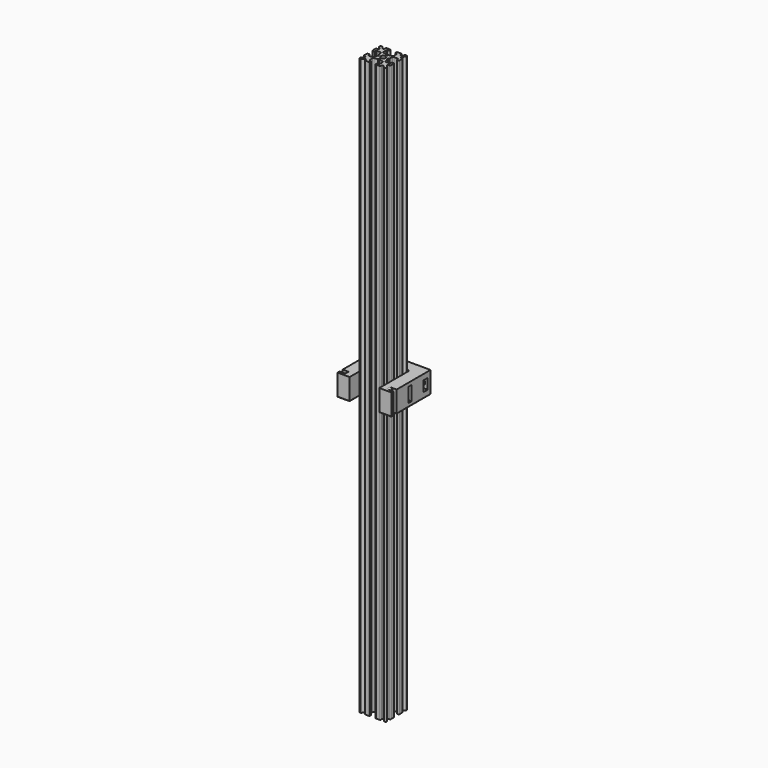
from build123d import *

# Parameters (mm, degrees)
F6_DEPTH  = 6
F7_DEPTH  = 160
F4_W      = 6
F4_H      = 2.8
F8_DEPTH  = 2.9
F11_DEPTH = 4
F12_R     = 1
F16_R     = 1.5
F13_SIZE  = 0.25


# Not quite as in the source:
# - a feature of the source that left no trace in its solid (it failed there, or was rolled back) is left out


with BuildPart() as f6:
    # F2 (on Top) → F6 (new body, symmetric)
    with BuildSketch(Plane.XY):
        Polygon((0, 14.1908953894), (-15, 14.1908953894), (-15, -9.4), (-12.8, -9.4), (-12.8, -11.6), (-15, -11.6), (-15, -13), (-8.25, -13), (-8.25, -8), (-8.25, 8), (8.25, 8), (8.25, -8), (8.25, -13), (15, -13), (15, -11.6), (12.8, -11.6), (12.8, -9.4), (15, -9.4), (15, 14.1908953894), align=None)
    extrude(amount=F6_DEPTH, both=True)

    # F4 (on Top) → F8 (cut, symmetric)
    with BuildSketch(Plane.XY):
        with Locations((-12, 10.7908953894)):
            Rectangle(F4_W, F4_H)
        with Locations((12, 10.7908953894)):
            Rectangle(F4_W, F4_H)
    extrude(amount=F8_DEPTH, both=True, mode=Mode.SUBTRACT)

    # F5 (on Top) → F9 (revolve, cut)
    with BuildSketch(Plane.XY):
        Polygon((-12, 7.8908953894), (-12, 12.1908953894), (-12, 14.1908953894), (-13.6, 14.1908953894), (-13.6, 12.1908953894), (-13.6, 7.8908953894), align=None)
    revolve(axis=Axis((-12, 13.1908953894, 0), (0, 1, 0)), mode=Mode.SUBTRACT)

    # F5 (on Top) → F10 (revolve, cut)
    with BuildSketch(Plane.XY):
        Polygon((12, 14.1908953894), (12, 12.1908953894), (12, 7.8908953894), (13.6, 7.8908953894), (13.6, 12.1908953894), (13.6, 14.1908953894), align=None)
    revolve(axis=Axis((12, 13.1908953894, 0), (0, 1, 0)), mode=Mode.SUBTRACT)

    # F3 (on Top) → F11 (cut, symmetric)
    with BuildSketch(Plane.XY):
        with BuildLine():
            ThreePointArc((-10.0158953894, 3.275), (-11.9460022518, 2.6458103674), (-13.1344888224, 1))
            Line((-13.1344888224, 1), (-21.4828029275, 1))
            Line((-21.4828029275, 1), (-21.4828029275, -1))
            Line((-21.4828029275, -1), (-13.1344888224, -1))
            ThreePointArc((-13.1344888224, -1), (-11.9460022518, -2.6458103674), (-10.0158953894, -3.275))
            Line((-10.0158953894, -3.275), (-8.25, -3.275))
            Line((-8.25, -3.275), (-8.25, 0))
            Line((-8.25, 0), (-8.25, 3.275))
            Line((-8.25, 3.275), (-10.0158953894, 3.275))
        make_face()
        with BuildLine():
            ThreePointArc((-1, 13.1344888224), (-2.6458103674, 11.9460022518), (-3.275, 10.0158953894))
            Line((-3.275, 10.0158953894), (-3.275, 8.25))
            Line((-3.275, 8.25), (0, 8.25))
            Line((0, 8.25), (3.275, 8.25))
            Line((3.275, 8.25), (3.275, 10.0158953894))
            ThreePointArc((3.275, 10.0158953894), (2.6458103674, 11.9460022518), (1, 13.1344888224))
            Line((1, 13.1344888224), (1, 21.4828029275))
            Line((1, 21.4828029275), (-1, 21.4828029275))
            Line((-1, 21.4828029275), (-1, 13.1344888224))
        make_face()
        Polygon((0, 8.25), (-3.275, 8.25), (-3.275, 2.3650461808), (3.275, 2.3650461808), (3.275, 8.25), align=None)
        with BuildLine():
            ThreePointArc((13.1344888224, 1), (11.9460022518, 2.6458103674), (10.0158953894, 3.275))
            Line((10.0158953894, 3.275), (8.25, 3.275))
            Line((8.25, 3.275), (8.25, 0))
            Line((8.25, 0), (8.25, -3.275))
            Line((8.25, -3.275), (10.0158953894, -3.275))
            ThreePointArc((10.0158953894, -3.275), (11.9460022518, -2.6458103674), (13.1344888224, -1))
            Line((13.1344888224, -1), (21.4828029275, -1))
            Line((21.4828029275, -1), (21.4828029275, 1))
            Line((21.4828029275, 1), (13.1344888224, 1))
        make_face()
    extrude(amount=F11_DEPTH, both=True, mode=Mode.SUBTRACT)

    # F12
    f12_edges = [f6.edges().sort_by_distance(p)[0] for p in [
        (-8.25, 8, 0),
        (8.25, 8, 0),
    ]]
    fillet(f12_edges, radius=F12_R)

    # F16
    f16_edges = [f6.edges().sort_by_distance(p)[0] for p in [
        (12.8, -10.5, -6),
        (-12.8, -10.5, -6),
        (12.8, -10.5, 6),
        (-12.8, -10.5, 6),
    ]]
    fillet(f16_edges, radius=F16_R)

    # F13
    f13_edges = [f6.edges().sort_by_distance(p)[0] for p in [
        (12.05, -11.6, -6),
        (13.9, -11.6, -6),
        (11.3, -10.5, -6),
        (15, -12.3, -6),
        (12.05, -9.4, -6),
        (11.625, -13, -6),
        (13.9, -9.4, -6),
        (8.25, -3, -6),
        (15, 2.395448, -6),
        (7.957107, 7.707107, -6),
        (0, 14.190895, -6),
        (0, 8, -6),
        (-15, 2.395448, -6),
        (-7.957107, 7.707107, -6),
        (-13.9, -9.4, -6),
        (-8.25, -3, -6),
        (-12.05, -9.4, -6),
        (-11.625, -13, -6),
        (-11.3, -10.5, -6),
        (-15, -12.3, -6),
        (-12.05, -11.6, -6),
        (-13.9, -11.6, -6),
    ]]
    chamfer(f13_edges, length=F13_SIZE)


with BuildPart() as f7:
    # F0 (on Top) → F7 (new body, symmetric)
    with BuildSketch(Plane.XY):
        with BuildLine():
            Line((-7.5, -6.7171572875), (-7.5, -7))
            ThreePointArc((-7.5, -7), (-7.3535533906, -7.3535533906), (-7, -7.5))
            Line((-7, -7.5), (-6.7171572875, -7.5))
            ThreePointArc((-6.7171572875, -7.5), (-6.5258155713, -7.4619397663), (-6.3636038969, -7.3535533906))
            Line((-6.3636038969, -7.3535533906), (-5.2564971157, -6.2464466094))
            ThreePointArc((-5.2564971157, -6.2464466094), (-4.711602009, -6.1380602337), (-4.4029437252, -6.6))
            Line((-4.4029437252, -6.6), (-4.4029437252, -7))
            ThreePointArc((-4.4029437252, -7), (-4.2564971157, -7.3535533906), (-3.9029437252, -7.5))
            Line((-3.9029437252, -7.5), (-2.1, -7.5))
            ThreePointArc((-2.1, -7.5), (-1.7464466094, -7.3535533906), (-1.6, -7))
            Line((-1.6, -7), (-1.6, -6.6))
            ThreePointArc((-1.6, -6.6), (-1.7464466094, -6.2464466094), (-2.1, -6.1))
            Line((-2.1, -6.1), (-2.7, -6.1))
            ThreePointArc((-2.7, -6.1), (-2.8414213562, -6.0414213562), (-2.9, -5.9))
            Line((-2.9, -5.9), (-2.9, -3.7379295017))
            ThreePointArc((-2.9, -3.7379295017), (-2.7836336902, -3.4172658278), (-2.4886992329, -3.2458599476))
            Line((-2.4886992329, -3.2458599476), (-0.7345203068, -2.929656021))
            ThreePointArc((-0.7345203068, -2.929656021), (-0.6165465239, -2.8610936689), (-0.57, -2.7328281993))
            Line((-0.57, -2.7328281993), (-0.57, -2.6))
            ThreePointArc((-0.57, -2.6), (-0.5114213562, -2.4585786438), (-0.37, -2.4))
            Line((-0.37, -2.4), (0, -2.4))
            Line((0, -2.4), (0.37, -2.4))
            ThreePointArc((0.37, -2.4), (0.5114213562, -2.4585786438), (0.57, -2.6))
            Line((0.57, -2.6), (0.57, -2.7328281993))
            ThreePointArc((0.57, -2.7328281993), (0.6165465239, -2.8610936689), (0.7345203068, -2.929656021))
            Line((0.7345203068, -2.929656021), (2.4886992329, -3.2458599476))
            ThreePointArc((2.4886992329, -3.2458599476), (2.7836336902, -3.4172658278), (2.9, -3.7379295017))
            Line((2.9, -3.7379295017), (2.9, -5.9))
            ThreePointArc((2.9, -5.9), (2.8414213562, -6.0414213562), (2.7, -6.1))
            Line((2.7, -6.1), (2.1, -6.1))
            ThreePointArc((2.1, -6.1), (1.7464466094, -6.2464466094), (1.6, -6.6))
            Line((1.6, -6.6), (1.6, -7))
            ThreePointArc((1.6, -7), (1.7464466094, -7.3535533906), (2.1, -7.5))
            Line((2.1, -7.5), (3.9029437252, -7.5))
            ThreePointArc((3.9029437252, -7.5), (4.2564971157, -7.3535533906), (4.4029437252, -7))
            Line((4.4029437252, -7), (4.4029437252, -6.6))
            ThreePointArc((4.4029437252, -6.6), (4.711602009, -6.1380602337), (5.2564971157, -6.2464466094))
            Line((5.2564971157, -6.2464466094), (6.3636038969, -7.3535533906))
            ThreePointArc((6.3636038969, -7.3535533906), (6.5258155713, -7.4619397663), (6.7171572875, -7.5))
            Line((6.7171572875, -7.5), (7, -7.5))
            ThreePointArc((7, -7.5), (7.3535533906, -7.3535533906), (7.5, -7))
            Line((7.5, -7), (7.5, -6.7171572875))
            ThreePointArc((7.5, -6.7171572875), (7.4619397663, -6.5258155713), (7.3535533906, -6.3636038969))
            Line((7.3535533906, -6.3636038969), (6.2464466094, -5.2564971157))
            ThreePointArc((6.2464466094, -5.2564971157), (6.1380602337, -4.711602009), (6.6, -4.4029437252))
            Line((6.6, -4.4029437252), (7, -4.4029437252))
            ThreePointArc((7, -4.4029437252), (7.3535533906, -4.2564971157), (7.5, -3.9029437252))
            Line((7.5, -3.9029437252), (7.5, -2.1))
            ThreePointArc((7.5, -2.1), (7.3535533906, -1.7464466094), (7, -1.6))
            Line((7, -1.6), (6.6, -1.6))
            ThreePointArc((6.6, -1.6), (6.2464466094, -1.7464466094), (6.1, -2.1))
            Line((6.1, -2.1), (6.1, -2.7))
            ThreePointArc((6.1, -2.7), (6.0414213562, -2.8414213562), (5.9, -2.9))
            Line((5.9, -2.9), (3.7379295017, -2.9))
            ThreePointArc((3.7379295017, -2.9), (3.4172658278, -2.7836336902), (3.2458599476, -2.4886992329))
            Line((3.2458599476, -2.4886992329), (2.929656021, -0.7345203068))
            ThreePointArc((2.929656021, -0.7345203068), (2.8610936689, -0.6165465239), (2.7328281993, -0.57))
            Line((2.7328281993, -0.57), (2.6, -0.57))
            ThreePointArc((2.6, -0.57), (2.4585786438, -0.5114213562), (2.4, -0.37))
            Line((2.4, -0.37), (2.4, 0))
            Line((2.4, 0), (2.4, 0.37))
            ThreePointArc((2.4, 0.37), (2.4585786438, 0.5114213562), (2.6, 0.57))
            Line((2.6, 0.57), (2.7328281993, 0.57))
            ThreePointArc((2.7328281993, 0.57), (2.8610936689, 0.6165465239), (2.929656021, 0.7345203068))
            Line((2.929656021, 0.7345203068), (3.2458599476, 2.4886992329))
            ThreePointArc((3.2458599476, 2.4886992329), (3.4172658278, 2.7836336902), (3.7379295017, 2.9))
            Line((3.7379295017, 2.9), (5.9, 2.9))
            ThreePointArc((5.9, 2.9), (6.0414213562, 2.8414213562), (6.1, 2.7))
            Line((6.1, 2.7), (6.1, 2.1))
            ThreePointArc((6.1, 2.1), (6.2464466094, 1.7464466094), (6.6, 1.6))
            Line((6.6, 1.6), (7, 1.6))
            ThreePointArc((7, 1.6), (7.3535533906, 1.7464466094), (7.5, 2.1))
            Line((7.5, 2.1), (7.5, 3.9029437252))
            ThreePointArc((7.5, 3.9029437252), (7.3535533906, 4.2564971157), (7, 4.4029437252))
            Line((7, 4.4029437252), (6.6, 4.4029437252))
            ThreePointArc((6.6, 4.4029437252), (6.1380602337, 4.711602009), (6.2464466094, 5.2564971157))
            Line((6.2464466094, 5.2564971157), (7.3535533906, 6.3636038969))
            ThreePointArc((7.3535533906, 6.3636038969), (7.4619397663, 6.5258155713), (7.5, 6.7171572875))
            Line((7.5, 6.7171572875), (7.5, 7))
            ThreePointArc((7.5, 7), (7.3535533906, 7.3535533906), (7, 7.5))
            Line((7, 7.5), (6.7171572875, 7.5))
            ThreePointArc((6.7171572875, 7.5), (6.5258155713, 7.4619397663), (6.3636038969, 7.3535533906))
            Line((6.3636038969, 7.3535533906), (5.2564971157, 6.2464466094))
            ThreePointArc((5.2564971157, 6.2464466094), (4.711602009, 6.1380602337), (4.4029437252, 6.6))
            Line((4.4029437252, 6.6), (4.4029437252, 7))
            ThreePointArc((4.4029437252, 7), (4.2564971157, 7.3535533906), (3.9029437252, 7.5))
            Line((3.9029437252, 7.5), (2.1, 7.5))
            ThreePointArc((2.1, 7.5), (1.7464466094, 7.3535533906), (1.6, 7))
            Line((1.6, 7), (1.6, 6.6))
            ThreePointArc((1.6, 6.6), (1.7464466094, 6.2464466094), (2.1, 6.1))
            Line((2.1, 6.1), (2.7, 6.1))
            ThreePointArc((2.7, 6.1), (2.8414213562, 6.0414213562), (2.9, 5.9))
            Line((2.9, 5.9), (2.9, 3.7379295017))
            ThreePointArc((2.9, 3.7379295017), (2.7836336902, 3.4172658278), (2.4886992329, 3.2458599476))
            Line((2.4886992329, 3.2458599476), (0.7345203068, 2.929656021))
            ThreePointArc((0.7345203068, 2.929656021), (0.6165465239, 2.8610936689), (0.57, 2.7328281993))
            Line((0.57, 2.7328281993), (0.57, 2.6))
            ThreePointArc((0.57, 2.6), (0.5114213562, 2.4585786438), (0.37, 2.4))
            Line((0.37, 2.4), (0, 2.4))
            Line((0, 2.4), (-0.37, 2.4))
            ThreePointArc((-0.37, 2.4), (-0.5114213562, 2.4585786438), (-0.57, 2.6))
            Line((-0.57, 2.6), (-0.57, 2.7328281993))
            ThreePointArc((-0.57, 2.7328281993), (-0.6165465239, 2.8610936689), (-0.7345203068, 2.929656021))
            Line((-0.7345203068, 2.929656021), (-2.4886992329, 3.2458599476))
            ThreePointArc((-2.4886992329, 3.2458599476), (-2.7836336902, 3.4172658278), (-2.9, 3.7379295017))
            Line((-2.9, 3.7379295017), (-2.9, 5.9))
            ThreePointArc((-2.9, 5.9), (-2.8414213562, 6.0414213562), (-2.7, 6.1))
            Line((-2.7, 6.1), (-2.1, 6.1))
            ThreePointArc((-2.1, 6.1), (-1.7464466094, 6.2464466094), (-1.6, 6.6))
            Line((-1.6, 6.6), (-1.6, 7))
            ThreePointArc((-1.6, 7), (-1.7464466094, 7.3535533906), (-2.1, 7.5))
            Line((-2.1, 7.5), (-3.9029437252, 7.5))
            ThreePointArc((-3.9029437252, 7.5), (-4.2564971157, 7.3535533906), (-4.4029437252, 7))
            Line((-4.4029437252, 7), (-4.4029437252, 6.6))
            ThreePointArc((-4.4029437252, 6.6), (-4.711602009, 6.1380602337), (-5.2564971157, 6.2464466094))
            Line((-5.2564971157, 6.2464466094), (-6.3636038969, 7.3535533906))
            ThreePointArc((-6.3636038969, 7.3535533906), (-6.5258155713, 7.4619397663), (-6.7171572875, 7.5))
            Line((-6.7171572875, 7.5), (-7, 7.5))
            ThreePointArc((-7, 7.5), (-7.3535533906, 7.3535533906), (-7.5, 7))
            Line((-7.5, 7), (-7.5, 6.7171572875))
            ThreePointArc((-7.5, 6.7171572875), (-7.4619397663, 6.5258155713), (-7.3535533906, 6.3636038969))
            Line((-7.3535533906, 6.3636038969), (-6.2464466094, 5.2564971157))
            ThreePointArc((-6.2464466094, 5.2564971157), (-6.1380602337, 4.711602009), (-6.6, 4.4029437252))
            Line((-6.6, 4.4029437252), (-7, 4.4029437252))
            ThreePointArc((-7, 4.4029437252), (-7.3535533906, 4.2564971157), (-7.5, 3.9029437252))
            Line((-7.5, 3.9029437252), (-7.5, 2.1))
            ThreePointArc((-7.5, 2.1), (-7.3535533906, 1.7464466094), (-7, 1.6))
            Line((-7, 1.6), (-6.6, 1.6))
            ThreePointArc((-6.6, 1.6), (-6.2464466094, 1.7464466094), (-6.1, 2.1))
            Line((-6.1, 2.1), (-6.1, 2.7))
            ThreePointArc((-6.1, 2.7), (-6.0414213562, 2.8414213562), (-5.9, 2.9))
            Line((-5.9, 2.9), (-3.7379295017, 2.9))
            ThreePointArc((-3.7379295017, 2.9), (-3.4172658278, 2.7836336902), (-3.2458599476, 2.4886992329))
            Line((-3.2458599476, 2.4886992329), (-2.929656021, 0.7345203068))
            ThreePointArc((-2.929656021, 0.7345203068), (-2.8610936689, 0.6165465239), (-2.7328281993, 0.57))
            Line((-2.7328281993, 0.57), (-2.6, 0.57))
            ThreePointArc((-2.6, 0.57), (-2.4585786438, 0.5114213562), (-2.4, 0.37))
            Line((-2.4, 0.37), (-2.4, 0))
            Line((-2.4, 0), (-2.4, -0.37))
            ThreePointArc((-2.4, -0.37), (-2.4585786438, -0.5114213562), (-2.6, -0.57))
            Line((-2.6, -0.57), (-2.7328281993, -0.57))
            ThreePointArc((-2.7328281993, -0.57), (-2.8610936689, -0.6165465239), (-2.929656021, -0.7345203068))
            Line((-2.929656021, -0.7345203068), (-3.2458599476, -2.4886992329))
            ThreePointArc((-3.2458599476, -2.4886992329), (-3.4172658278, -2.7836336902), (-3.7379295017, -2.9))
            Line((-3.7379295017, -2.9), (-5.9, -2.9))
            ThreePointArc((-5.9, -2.9), (-6.0414213562, -2.8414213562), (-6.1, -2.7))
            Line((-6.1, -2.7), (-6.1, -2.1))
            ThreePointArc((-6.1, -2.1), (-6.2464466094, -1.7464466094), (-6.6, -1.6))
            Line((-6.6, -1.6), (-7, -1.6))
            ThreePointArc((-7, -1.6), (-7.3535533906, -1.7464466094), (-7.5, -2.1))
            Line((-7.5, -2.1), (-7.5, -3.9029437252))
            ThreePointArc((-7.5, -3.9029437252), (-7.3535533906, -4.2564971157), (-7, -4.4029437252))
            Line((-7, -4.4029437252), (-6.6, -4.4029437252))
            ThreePointArc((-6.6, -4.4029437252), (-6.1380602337, -4.711602009), (-6.2464466094, -5.2564971157))
            Line((-6.2464466094, -5.2564971157), (-7.3535533906, -6.3636038969))
            ThreePointArc((-7.3535533906, -6.3636038969), (-7.4619397663, -6.5258155713), (-7.5, -6.7171572875))
        make_face()
        with BuildLine():
            ThreePointArc((-0.9545941546, -0.9545941546), (-1.2472373689, -0.5166226337), (-1.35, 0))
            ThreePointArc((-1.35, 0), (-1.2472373689, 0.5166226337), (-0.9545941546, 0.9545941546))
            ThreePointArc((-0.9545941546, 0.9545941546), (-0.5166226337, 1.2472373689), (0, 1.35))
            ThreePointArc((0, 1.35), (0.5166226337, 1.2472373689), (0.9545941546, 0.9545941546))
            ThreePointArc((0.9545941546, 0.9545941546), (1.2472373689, 0.5166226337), (1.35, 0))
            ThreePointArc((1.35, 0), (1.2472373689, -0.5166226337), (0.9545941546, -0.9545941546))
            ThreePointArc((0.9545941546, -0.9545941546), (0.5166226337, -1.2472373689), (0, -1.35))
            ThreePointArc((0, -1.35), (-0.5166226337, -1.2472373689), (-0.9545941546, -0.9545941546))
        make_face(mode=Mode.SUBTRACT)
    extrude(amount=F7_DEPTH, both=True)


solid = Compound([f6.part, f7.part])
